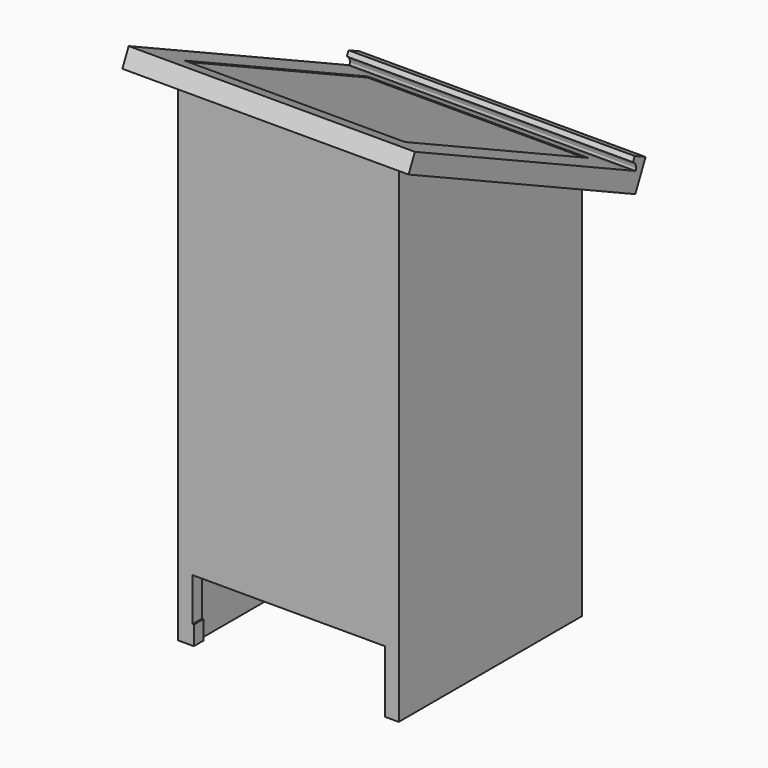
from build123d import *

# Parameters (mm, degrees)
F1_DEPTH    = 47.4263094366
F2_W        = 61.5427512676
F2_H        = 67.2771147457
F2_W_2      = 47.4263094366
F2_H_2      = 54.3905875297
F3_DEPTH    = 3.989492543
F4_DEPTH    = 3.7897219881
F5_W        = 61.5427512676
F5_H        = 3.2427412463
F6_DEPTH    = 2.5458927266
F7_W        = 41.3791541941
F7_H        = 73.2382405549
F8_DEPTH    = 1.1647148058
F9_T        = 2.54
F9_T3_DEPTH = 6.2447148058
F9_T5_DEPTH = 78.3182405549
F9_T7_DEPTH = 46.4591541941
F10_W       = 41.3791541941
F10_H       = 9.277254343
F11_DEPTH   = 51.4699444175
F12_W       = 41.0984121263
F12_H       = 4.0935091674
F13_DEPTH   = 56.4465969801
F14_W       = 3.1205418054
F14_H       = 6.5310224891
F14_W_2     = 3.1721270643
F15_DEPTH   = 43.8657402992
F16_W       = 39.7140569985
F16_H       = 81.2445171177
F17_DEPTH   = 10
F19_DEPTH   = 80.7498022914


# Not quite as in the source:
# - a shell that OpenCascade refuses in one call is made with other operations: the cavity is built on its own and cut out


with BuildPart() as f1:
    # F0 (on Right) → F1 (new body)
    with BuildSketch(Plane.YZ):
        Polygon((24.6358662844, 29.6986699104), (-24.6358662844, 52.7341291308), (-24.6358662844, -52.7341291308), (24.6358662844, -52.7341291308), align=None)
    extrude(amount=F1_DEPTH)


with BuildPart() as f3:
    # F2 (on face) → F3 (new body)
    with BuildSketch(Plane(origin=(0, 15.8131088069, 33.8234745294), x_dir=(1, 0, 0), z_dir=(0, 0.4235192203, 0.9058871177))):
        with Locations((23.4371926636, -17.4559373872)):
            Rectangle(F2_W, F2_H)
        with Locations((23.7131547183, -17.4559373872)):
            Rectangle(F2_W_2, F2_H_2, mode=Mode.SUBTRACT)
    extrude(amount=F3_DEPTH)

    # F5 (on face) → F6 (join)
    with BuildSketch(Plane(origin=(0, 17.502735578, 37.4375044304), x_dir=(1, 0, 0), z_dir=(0, 0.4235192203, 0.9058871177))):
        with Locations((23.4371926636, 14.5612493625)):
            Rectangle(F5_W, F5_H)
    extrude(amount=F6_DEPTH)

    # F18 (on face) → F19 (cut)
    with BuildSketch(Plane.YZ.offset(54.2085682973)):
        with BuildLine():
            Line((29.224805033, 31.9572170763), (30.5427146714, 31.3410695989))
            ThreePointArc((30.5427146714, 31.3410695989), (30.6449907476, 31.6416286341), (30.6796326959, 31.9572170763))
            ThreePointArc((30.6796326959, 31.9572170763), (30.4521827099, 32.7382852981), (29.8409525104, 33.2751267147))
            Line((29.8409525104, 33.2751267147), (29.224805033, 31.9572170763))
        make_face()
    extrude(amount=-F19_DEPTH, mode=Mode.SUBTRACT)


with BuildPart() as f4:
    # F4 (new): a face of the model
    f4_faces = [f1.part.faces().sort_by_distance(p)[0] for p in [
        (23.7131547183, 0, 41.2163995206),
    ]]
    extrude(f4_faces, amount=F4_DEPTH)


with BuildPart() as f1_1:
    add(f1.part)

    # F7 (on face) → F8 (cut)
    with BuildSketch(Plane(origin=(0, 24.6358662844, 0), x_dir=(-1, 0, 0), z_dir=(0, 1, 0))):
        with Locations((-23.7684322055, -12.0214996859)):
            Rectangle(F7_W, F7_H)
    extrude(amount=-F8_DEPTH, mode=Mode.SUBTRACT)

    # F9: shell of thickness 2.54, made by hand


with BuildPart() as f9_core1:
    # F9_t2: copy of F1
    add(f1_1.part)

    # the walls: a layer under each face that stays
    f9_faces = [f9_core1.faces().sort_by_distance(p)[0] for p in [
        (23.7131547183, 0, 41.2163995206),
        (45.8454324553, 24.6358662844, -49.9863691628),
        (23.7131547183, -24.6358662844, 0),
        (0, 0, 0),
        (47.4263094366, 0, 0),
        (3.0788551085, 24.0535088815, -12.0214996859),
        (23.7684322055, 24.0535088815, -48.6406199634),
        (44.4580093026, 24.0535088815, -12.0214996859),
        (23.7684322055, 24.0535088815, 24.5976205915),
        (23.7684322055, 23.4711514786, -12.0214996859),
    ]]
    thicken(f9_faces, amount=-F9_T, mode=Mode.SUBTRACT)

    # F9_s4 → F9_t3 (cut)
    with BuildSketch(Plane.XZ.offset(-27.1758662844)):
        Polygon((3.1042551085, -48.6152199634), (0.5388551085, -48.6406199634), (0.5388551085, -51.1806199634), (3.0788551085, -51.1806199634), align=None)
        Polygon((3.1042551085, 24.5722205915), (0.5388551085, 24.5976205915), (0.5388551085, 27.1376205915), (3.0788551085, 27.1376205915), align=None)
        Polygon((44.4326093026, -48.6152199634), (44.4580093026, -51.1806199634), (46.9980093026, -51.1806199634), (46.9980093026, -48.6406199634), align=None)
        Polygon((44.4326093026, 24.5722205915), (46.9980093026, 24.5976205915), (46.9980093026, 27.1376205915), (44.4580093026, 27.1376205915), align=None)
    extrude(amount=F9_T3_DEPTH, mode=Mode.SUBTRACT)

    # F9_s6 → F9_t5 (cut)
    with BuildSketch(Plane.XY.offset(-51.1806199634)):
        Polygon((3.1042551085, 23.4965514786), (0.5388551085, 23.4711514786), (0.5388551085, 20.9311514786), (3.0788551085, 20.9311514786), align=None)
        Polygon((44.4326093026, 23.4965514786), (46.9980093026, 23.4711514786), (46.9980093026, 20.9311514786), (44.4580093026, 20.9311514786), align=None)
    extrude(amount=F9_T5_DEPTH, mode=Mode.SUBTRACT)

    # F9_s8 → F9_t7 (cut)
    with BuildSketch(Plane.YZ.offset(0.5388551085)):
        Polygon((23.4965514786, -48.6152199634), (23.4711514786, -51.1806199634), (20.9311514786, -51.1806199634), (20.9311514786, -48.6406199634), align=None)
        Polygon((23.4965514786, 24.5722205915), (23.4711514786, 27.1376205915), (20.9311514786, 27.1376205915), (20.9311514786, 24.5976205915), align=None)
    extrude(amount=F9_T7_DEPTH, mode=Mode.SUBTRACT)


with BuildPart() as f1_2:
    add(f1_1.part)

    # what is left inside the walls is the cavity
    f9_cavity = [f9_core1.part.solids().sort_by_distance(p)[0] for p in [
        (30.770873, -22.070466, -1.99569),
    ]]
    add(f9_cavity, mode=Mode.SUBTRACT)

    # F10 (on face) → F11 (cut)
    with BuildSketch(Plane(origin=(0, 23.4711514786, 0), x_dir=(-1, 0, 0), z_dir=(0, 1, 0))):
        with Locations((-23.7684322055, -44.0019927919)):
            Rectangle(F10_W, F10_H)
    extrude(amount=-F11_DEPTH, mode=Mode.SUBTRACT)

    # F12 (on face) → F13 (cut)
    with BuildSketch(Plane(origin=(0, 24.6358662844, 0), x_dir=(-1, 0, 0), z_dir=(0, 1, 0))):
        with Locations((-23.9088032395, -50.6873745471)):
            Rectangle(F12_W, F12_H)
    extrude(amount=-F13_DEPTH, mode=Mode.SUBTRACT)

    # F14 (on face) → F15 (join)
    with BuildSketch(Plane.YZ.offset(2.54)):
        with Locations((-1.5602709027, -39.8372523487)):
            Rectangle(F14_W, F14_H)
        with Locations((1.5860635322, -39.8372523487)):
            Rectangle(F14_W_2, F14_H)
    extrude(amount=F15_DEPTH)

    # F16 (on face) → F17 (cut)
    with BuildSketch(Plane.XZ.offset(24.6358662844)):
        with Locations((22.683288902, 4.934841767)):
            Rectangle(F16_W, F16_H)
    extrude(amount=F17_DEPTH, mode=Mode.SUBTRACT)


solid = Compound([f3.part, f4.part, f1_2.part])
